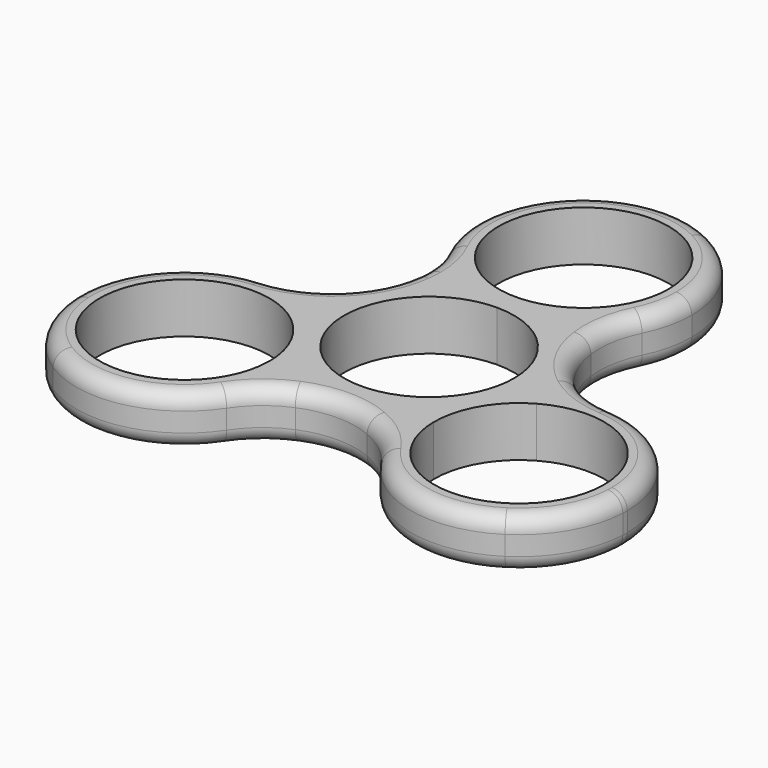
from build123d import *

# Parameters (mm, degrees)
F1_DEPTH = 6.5
F2_R     = 2


# Not quite as in the source:
# - a feature names something its author has since deleted; it is built from what else it names


with BuildPart() as f1:
    # F0 (on Top) → F1 (new body)
    with BuildSketch(Plane.XY):
        with BuildLine():
            ThreePointArc((6.3834473445, 37.46), (0, 39), (-6.3834473445, 37.46))
            ThreePointArc((-6.3834473445, 37.46), (0, 38), (6.3834473445, 37.46))
        make_face()
        with BuildLine():
            ThreePointArc((-12.5422634057, 18.7797404667), (-10.8800030067, 16.1894645694), (-8.6919143461, 14.025))
            ThreePointArc((-8.6919143461, 14.025), (-7.1791791885, 14.8562911313), (-5.587877504, 15.525))
            ThreePointArc((-5.587877504, 15.525), (-5.4558843213, 34.5516138046), (11, 25))
            ThreePointArc((11, 25), (9.5516138046, 19.5441156787), (5.587877504, 15.525))
            ThreePointArc((5.587877504, 15.525), (7.1791791885, 14.8562911313), (8.6919143461, 14.025))
            ThreePointArc((8.6919143461, 14.025), (10.8800030203, 16.1894645861), (12.5422634249, 18.7797405054))
            ThreePointArc((12.5422634249, 18.7797405054), (13.630694919, 21.8056055307), (14, 25))
            ThreePointArc((14, 25), (11.9450463127, 32.3017716062), (6.3834473445, 37.46))
            ThreePointArc((6.3834473445, 37.46), (0, 38), (-6.3834473445, 37.46))
            ThreePointArc((-6.3834473445, 37.46), (-13.2960015008, 29.3836450691), (-12.5422634057, 18.7797404667))
        make_face()
        with BuildLine():
            ThreePointArc((-9.5262796431, -5.499999651), (-9.5262793442, 5.5000001687), (-1.34e-08, 11))
            ThreePointArc((-1.34e-08, 11), (-4.6016301523, 11.7778594796), (-8.6919143461, 14.025))
            ThreePointArc((-8.6919143461, 14.025), (-10.0938848824, 13.0523364951), (-11.3879056975, 11.940083912))
            ThreePointArc((-11.3879056975, 11.940083912), (-12.9004703417, 7.4480900244), (-16.0343688398, 3.8921736739))
            ThreePointArc((-16.0343688398, 3.8921736739), (-16.3505974247, 2.2153924835), (-16.4919634611, 0.5149186312))
            ThreePointArc((-16.4919634611, 0.5149186312), (-12.5007407351, -1.9038010018), (-9.5262796431, -5.499999651))
        make_face()
        with BuildLine():
            ThreePointArc((-1.34e-08, 11), (7.7781745883, 7.7781745978), (11, 0))
            ThreePointArc((11, 0), (10.6251841562, -2.8470092462), (9.5262797004, -5.4999995518))
            ThreePointArc((9.5262797004, -5.4999995518), (12.5007407784, -1.9038009644), (16.4919634611, 0.5149186312))
            ThreePointArc((16.4919634611, 0.5149186312), (16.3505974247, 2.2153924835), (16.0343688398, 3.8921736739))
            ThreePointArc((16.0343688398, 3.8921736739), (12.9004703417, 7.4480900244), (11.3879056975, 11.940083912))
            ThreePointArc((11.3879056975, 11.940083912), (10.0938848824, 13.0523364951), (8.6919143461, 14.025))
            ThreePointArc((8.6919143461, 14.025), (4.6016301396, 11.7778594752), (-1.34e-08, 11))
        make_face()
        with BuildLine():
            ThreePointArc((7.800049115, -14.5399186312), (7.8991104852, -9.8740580897), (9.5262797004, -5.4999995518))
            ThreePointArc((9.5262797004, -5.4999995518), (5.73e-08, -11), (-9.5262796431, -5.499999651))
            ThreePointArc((-9.5262796431, -5.499999651), (-8.1276735787, -8.876533174), (-7.6506350946, -12.5))
            ThreePointArc((-7.6506350946, -12.5), (-7.6880385647, -13.5226916167), (-7.800049115, -14.5399186312))
            ThreePointArc((-7.800049115, -14.5399186312), (-6.2567125423, -15.2677289786), (-4.6464631424, -15.8322575859))
            ThreePointArc((-4.6464631424, -15.8322575859), (0, -14.8961800489), (4.6464631424, -15.8322575859))
            ThreePointArc((4.6464631424, -15.8322575859), (6.2567125423, -15.2677289786), (7.800049115, -14.5399186312))
        make_face()
        with BuildLine():
            ThreePointArc((-16.2389831458, -2.9232561283), (-16.45551512, -1.2107940101), (-16.4919634611, 0.5149186312))
            ThreePointArc((-16.4919634611, 0.5149186312), (-19.4604892606, 1.3276267387), (-22.53486436, 1.4720484757))
            ThreePointArc((-22.53486436, 1.4720484757), (-32.0949839483, -3.1771475919), (-35.633035298, -13.2017724359))
            ThreePointArc((-35.633035298, -13.2017724359), (-32.9089653438, -19), (-29.2495879535, -24.2582275641))
            ThreePointArc((-29.2495879535, -24.2582275641), (-18.7989825271, -26.2064976429), (-9.9926008348, -20.25178929))
            ThreePointArc((-9.9926008348, -20.25178929), (-8.5804861576, -17.5170914646), (-7.800049115, -14.5399186312))
            ThreePointArc((-7.800049115, -14.5399186312), (-9.2763359315, -13.6454971212), (-10.6511056417, -12.6017438717))
            ThreePointArc((-10.6511056417, -12.6017438717), (-31.1769145362, -18), (-16.2389831458, -2.9232561283))
        make_face()
        with BuildLine():
            ThreePointArc((-29.2495879535, -24.2582275641), (-32.9089653438, -19), (-35.633035298, -13.2017724359))
            ThreePointArc((-35.633035298, -13.2017724359), (-33.7749907476, -19.5), (-29.2495879535, -24.2582275641))
        make_face()
        with BuildLine():
            ThreePointArc((22.5348640827, 1.4720484932), (19.4604891234, 1.327626717), (16.4919634611, 0.5149186312))
            ThreePointArc((16.4919634611, 0.5149186312), (16.4979907429, 0.2574906711), (16.5, 0))
            ThreePointArc((16.5, 0), (16.4346162399, -1.4674430304), (16.2389831458, -2.9232561283))
            ThreePointArc((16.2389831458, -2.9232561283), (27.1946331359, -2.9992586753), (32.6506350946, -12.5))
            ThreePointArc((32.6506350946, -12.5), (21.7015075745, -23.4998823626), (10.6511056417, -12.6017438717))
            ThreePointArc((10.6511056417, -12.6017438717), (9.2763359315, -13.6454971212), (7.800049115, -14.5399186312))
            ThreePointArc((7.800049115, -14.5399186312), (8.580486101, -17.5170913173), (9.9926006599, -20.2517890271))
            ThreePointArc((9.9926006599, -20.2517890271), (18.7989823725, -26.2064976107), (29.2495879535, -24.2582275641))
            ThreePointArc((29.2495879535, -24.2582275641), (32.9089653438, -19), (35.633035298, -13.2017724359))
            ThreePointArc((35.633035298, -13.2017724359), (35.6462344538, -12.8509965472), (35.6506350946, -12.5))
            ThreePointArc((35.6506350946, -12.5), (31.8579659366, -2.9182257863), (22.5348640827, 1.4720484932))
        make_face()
        with BuildLine():
            ThreePointArc((35.633035298, -13.2017724359), (32.9089653438, -19), (29.2495879535, -24.2582275641))
            ThreePointArc((29.2495879535, -24.2582275641), (33.7749907476, -19.5), (35.633035298, -13.2017724359))
        make_face()
        with BuildLine():
            ThreePointArc((12.5422634249, 18.7797405054), (10.8800030203, 16.1894645861), (8.6919143461, 14.025))
            ThreePointArc((8.6919143461, 14.025), (10.0938848824, 13.0523364951), (11.3879056975, 11.940083912))
            ThreePointArc((11.3879056975, 11.940083912), (11.4601169695, 15.4451377216), (12.5422634249, 18.7797405054))
        make_face()
        with BuildLine():
            ThreePointArc((-11.3879056975, 11.940083912), (-10.0938848824, 13.0523364951), (-8.6919143461, 14.025))
            ThreePointArc((-8.6919143461, 14.025), (-10.8800030067, 16.1894645694), (-12.5422634057, 18.7797404667))
            ThreePointArc((-12.5422634057, 18.7797404667), (-11.609322329, 16.1861421262), (-11.2927751871, 13.4480900244))
            ThreePointArc((-11.2927751871, 13.4480900244), (-11.3165814287, 12.6925881632), (-11.3879056975, 11.940083912))
        make_face()
        with BuildLine():
            ThreePointArc((-4.6464631424, -15.8322575859), (-6.2567125423, -15.2677289786), (-7.800049115, -14.5399186312))
            ThreePointArc((-7.800049115, -14.5399186312), (-8.5804861576, -17.5170914646), (-9.9926008348, -20.25178929))
            ThreePointArc((-9.9926008348, -20.25178929), (-7.6458232815, -17.6473213978), (-4.6464631424, -15.8322575859))
        make_face()
        with BuildLine():
            ThreePointArc((-7.6506350946, -12.5), (-8.1276735787, -8.876533174), (-9.5262796431, -5.499999651))
            ThreePointArc((-9.5262796431, -5.499999651), (-12.5007407351, -1.9038010018), (-16.4919634611, 0.5149186312))
            ThreePointArc((-16.4919634611, 0.5149186312), (-16.45551512, -1.2107940101), (-16.2389831458, -2.9232561283))
            ThreePointArc((-16.2389831458, -2.9232561283), (-12.1498937699, -6.9560019588), (-10.6506350946, -12.5))
            ThreePointArc((-10.6506350946, -12.5), (-10.650752732, -12.5508724799), (-10.6511056417, -12.6017438717))
            ThreePointArc((-10.6511056417, -12.6017438717), (-9.2763359315, -13.6454971212), (-7.800049115, -14.5399186312))
            ThreePointArc((-7.800049115, -14.5399186312), (-7.6880385647, -13.5226916167), (-7.6506350946, -12.5))
        make_face()
        with BuildLine():
            ThreePointArc((-8.6919143461, 14.025), (-4.6016301523, 11.7778594796), (-1.34e-08, 11))
            ThreePointArc((-1.34e-08, 11), (4.6016301396, 11.7778594752), (8.6919143461, 14.025))
            ThreePointArc((8.6919143461, 14.025), (7.1791791885, 14.8562911313), (5.587877504, 15.525))
            ThreePointArc((5.587877504, 15.525), (0, 14), (-5.587877504, 15.525))
            ThreePointArc((-5.587877504, 15.525), (-7.1791791885, 14.8562911313), (-8.6919143461, 14.025))
        make_face()
        with BuildLine():
            ThreePointArc((16.4919634611, 0.5149186312), (12.5007407784, -1.9038009644), (9.5262797004, -5.4999995518))
            ThreePointArc((9.5262797004, -5.4999995518), (7.8991104852, -9.8740580897), (7.800049115, -14.5399186312))
            ThreePointArc((7.800049115, -14.5399186312), (9.2763359315, -13.6454971212), (10.6511056417, -12.6017438717))
            ThreePointArc((10.6511056417, -12.6017438717), (12.124355653, -7), (16.2389831458, -2.9232561283))
            ThreePointArc((16.2389831458, -2.9232561283), (16.4346162399, -1.4674430304), (16.5, 0))
            ThreePointArc((16.5, 0), (16.4979907429, 0.2574906711), (16.4919634611, 0.5149186312))
        make_face()
        with BuildLine():
            ThreePointArc((16.0343688398, 3.8921736739), (16.3505974247, 2.2153924835), (16.4919634611, 0.5149186312))
            ThreePointArc((16.4919634611, 0.5149186312), (19.4604891234, 1.327626717), (22.5348640827, 1.4720484932))
            ThreePointArc((22.5348640827, 1.4720484932), (19.1059401242, 2.2021835623), (16.0343688398, 3.8921736739))
        make_face()
        with BuildLine():
            ThreePointArc((-22.53486436, 1.4720484757), (-19.4604892606, 1.3276267387), (-16.4919634611, 0.5149186312))
            ThreePointArc((-16.4919634611, 0.5149186312), (-16.3505974247, 2.2153924835), (-16.0343688398, 3.8921736739))
            ThreePointArc((-16.0343688398, 3.8921736739), (-19.1059402544, 2.2021835138), (-22.53486436, 1.4720484757))
        make_face()
        with BuildLine():
            ThreePointArc((9.9926006599, -20.2517890271), (8.580486101, -17.5170913173), (7.800049115, -14.5399186312))
            ThreePointArc((7.800049115, -14.5399186312), (6.2567125423, -15.2677289786), (4.6464631424, -15.8322575859))
            ThreePointArc((4.6464631424, -15.8322575859), (7.6458231599, -17.6473212972), (9.9926006599, -20.2517890271))
        make_face()
    extrude(amount=F1_DEPTH)

    # F2
    f2_edges = [f1.edges().sort_by_distance(p)[0] for p in [
        (0, 39, 6.5),
        (0, 39, 0),
        (33.774991, -19.5, 0),
        (33.774991, -19.5, 6.5),
        (12.90047, 7.44809, 0),
        (12.90047, 7.44809, 6.5),
        (-12.90047, 7.44809, 0),
        (-12.90047, 7.44809, 6.5),
        (-33.774991, -19.5, 0),
        (-33.774991, -19.5, 6.5),
        (0, -14.89618, 0),
        (0, -14.89618, 6.5),
    ]]
    fillet(f2_edges, radius=F2_R)


solid = f1.part
